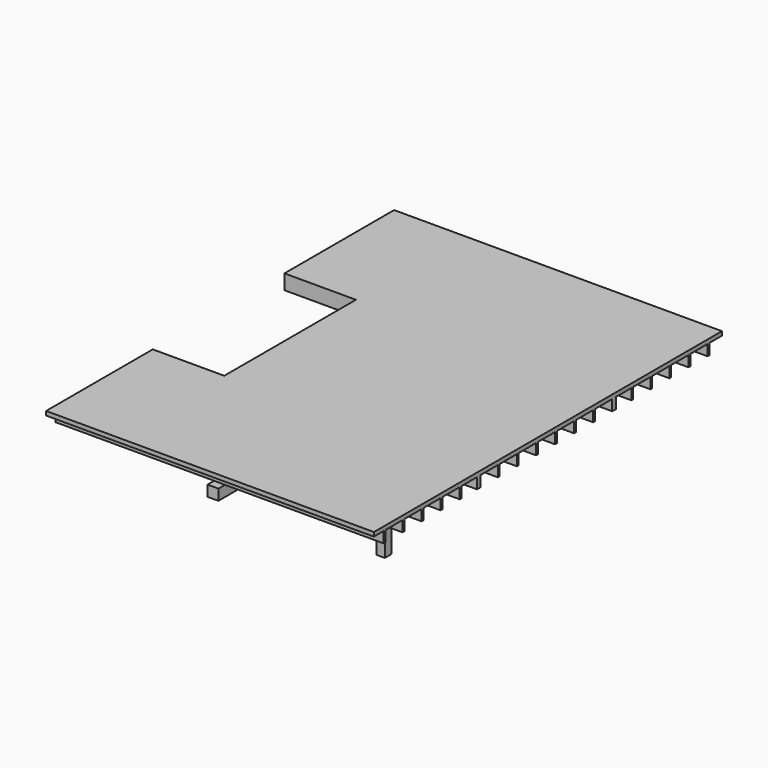
from build123d import *

# Parameters (mm, degrees)
F0_W      = 5867.4
F0_H      = 7696.2
F1_DEPTH  = 69.135625
F2_W      = 5867.4
F2_H      = 7696.2
F2_W_2    = 5791.2
F2_H_2    = 7620
F3_DEPTH  = 184.15
F4_W      = 38.1
F4_H      = 184.15
F5_DEPTH  = 5863.2060388453
F7_W      = 184.15
F7_H      = 184.15
F8_DEPTH  = 7289.8
F9_W      = 139.7
F9_H      = 139.7
F10_DEPTH = 2317.62046
F12_DEPTH = 139.7
F13_W     = 5867.4
F13_H     = 7696.2
F13_W_2   = 5590.8448
F13_H_2   = 7419.6448
F14_DEPTH = 253.285625
F15_W     = 1219.2
F15_H     = 2806.7
F16_DEPTH = 253.285625
F17_W     = 368.3
F17_H     = 184.15
F18_DEPTH = 38.1
F19_DEPTH = 38.1
F20_DEPTH = 38.1


with BuildPart() as f1:
    # F0 (on Top) → F1 (new body)
    with BuildSketch(Plane.XY):
        with Locations((2929.5060388453, -3848.1)):
            Rectangle(F0_W, F0_H)
    extrude(amount=F1_DEPTH)

    # F2 (on face) → F3 (join)
    with BuildSketch(Plane(origin=(0, 0, 0), x_dir=(1, 0, 0), z_dir=(0, 0, -1))):
        with Locations((2929.5060388453, 3848.1)):
            Rectangle(F2_W, F2_H)
        with Locations((2929.5060388453, 3848.1)):
            Rectangle(F2_W_2, F2_H_2, mode=Mode.SUBTRACT)
    extrude(amount=F3_DEPTH)

    # F4 (on Right) → F5 (join, through all)
    with BuildSketch(Plane.YZ):
        with Locations((-425.45, -92.075)):
            Rectangle(F4_W, F4_H)
        with Locations((-831.85, -92.075)):
            Rectangle(F4_W, F4_H)
        with Locations((-1238.25, -92.075)):
            Rectangle(F4_W, F4_H)
        with Locations((-1644.65, -92.075)):
            Rectangle(F4_W, F4_H)
        with Locations((-2051.05, -92.075)):
            Rectangle(F4_W, F4_H)
        with Locations((-2457.45, -92.075)):
            Rectangle(F4_W, F4_H)
        with Locations((-2863.85, -92.075)):
            Rectangle(F4_W, F4_H)
        with Locations((-3270.25, -92.075)):
            Rectangle(F4_W, F4_H)
        with Locations((-3676.65, -92.075)):
            Rectangle(F4_W, F4_H)
        with Locations((-4083.05, -92.075)):
            Rectangle(F4_W, F4_H)
        with Locations((-4489.45, -92.075)):
            Rectangle(F4_W, F4_H)
        with Locations((-4895.85, -92.075)):
            Rectangle(F4_W, F4_H)
        with Locations((-5302.25, -92.075)):
            Rectangle(F4_W, F4_H)
        with Locations((-5708.65, -92.075)):
            Rectangle(F4_W, F4_H)
        with Locations((-6115.05, -92.075)):
            Rectangle(F4_W, F4_H)
        with Locations((-6521.45, -92.075)):
            Rectangle(F4_W, F4_H)
        with Locations((-6927.85, -92.075)):
            Rectangle(F4_W, F4_H)
        with Locations((-7334.25, -92.075)):
            Rectangle(F4_W, F4_H)
    extrude(amount=F5_DEPTH)

    # F7 (on offset) → F8 (join)
    with BuildSketch(Plane(origin=(0, -203.2, 0), x_dir=(-1, 0, 0), z_dir=(0, 1, 0))):
        with Locations((-2929.5060388453, -276.225)):
            Rectangle(F7_W, F7_H)
    extrude(amount=-F8_DEPTH)

    # F9 (on face) → F10 (join)
    with BuildSketch(Plane(origin=(0, 0, -368.3), x_dir=(1, 0, 0), z_dir=(0, 0, -1))):
        with Locations((2929.5060388453, 3848.1)):
            Rectangle(F9_W, F9_H)
    extrude(amount=F10_DEPTH)

    # F11 (on face) → F12 (join, through all)
    with BuildSketch(Plane.YZ.offset(2999.3560388453)):
        Polygon((-3917.95, -780.3343653365), (-4329.9843653365, -368.3), (-4527.55, -368.3), (-3917.95, -977.9), align=None)
        Polygon((-3366.2156346635, -368.3), (-3778.25, -780.3343653365), (-3778.25, -977.9), (-3168.65, -368.3), align=None)
    extrude(amount=-F12_DEPTH)

    # F13 (on face) → F14 (cut, through all)
    with BuildSketch(Plane.XY.offset(69.135625)):
        with Locations((2929.5060388453, -3848.1)):
            Rectangle(F13_W, F13_H)
        with Locations((2929.5060388453, -3848.1)):
            Rectangle(F13_W_2, F13_H_2, mode=Mode.SUBTRACT)
    extrude(amount=-F14_DEPTH, mode=Mode.SUBTRACT)

    # F15 (on face) → F16 (cut, through all)
    with BuildSketch(Plane.XY.offset(69.135625)):
        with Locations((743.6836388453, -3879.85)):
            Rectangle(F15_W, F15_H)
    extrude(amount=-F16_DEPTH, mode=Mode.SUBTRACT)

    # F17 (on face) → F18 (join)
    with BuildSketch(Plane(origin=(1353.2836388453, 0, 0), x_dir=(0, -1, 0), z_dir=(-1, 0, 0))):
        Polygon((5283.2, 69.135625), (2476.5, 69.135625), (2476.5, 0), (2844.8, 0), (2844.8, -184.15), (2882.9, -184.15), (2882.9, 0), (3251.2, 0), (3251.2, -184.15), (3289.3, -184.15), (3289.3, 0), (3657.6, 0), (3657.6, -184.15), (3695.7, -184.15), (3695.7, 0), (4064, 0), (4064, -184.15), (4102.1, -184.15), (4102.1, 0), (4470.4, 0), (4470.4, -184.15), (4508.5, -184.15), (4508.5, 0), (4876.8, 0), (4876.8, -184.15), (4914.9, -184.15), (4914.9, 0), (5283.2, 0), align=None)
        with Locations((2660.65, -92.075)):
            Rectangle(F17_W, F17_H)
        with Locations((5099.05, -92.075)):
            Rectangle(F17_W, F17_H)
        with Locations((3067.05, -92.075)):
            Rectangle(F17_W, F17_H)
        with Locations((4692.65, -92.075)):
            Rectangle(F17_W, F17_H)
        with Locations((3473.45, -92.075)):
            Rectangle(F17_W, F17_H)
        with Locations((4286.25, -92.075)):
            Rectangle(F17_W, F17_H)
        with Locations((3879.85, -92.075)):
            Rectangle(F17_W, F17_H)
    extrude(amount=-F18_DEPTH)

    # F19 (add): a face of the model
    f19_faces = [f1.faces().sort_by_distance(p)[0] for p in [
        (2929.5060388453, -5321.3, -92.075),
    ]]
    extrude(f19_faces, amount=F19_DEPTH)

    # F20 (add): a face of the model
    f20_faces = [f1.faces().sort_by_distance(p)[0] for p in [
        (2929.5060388453, -2438.4, -92.075),
    ]]
    extrude(f20_faces, amount=F20_DEPTH)


solid = f1.part
